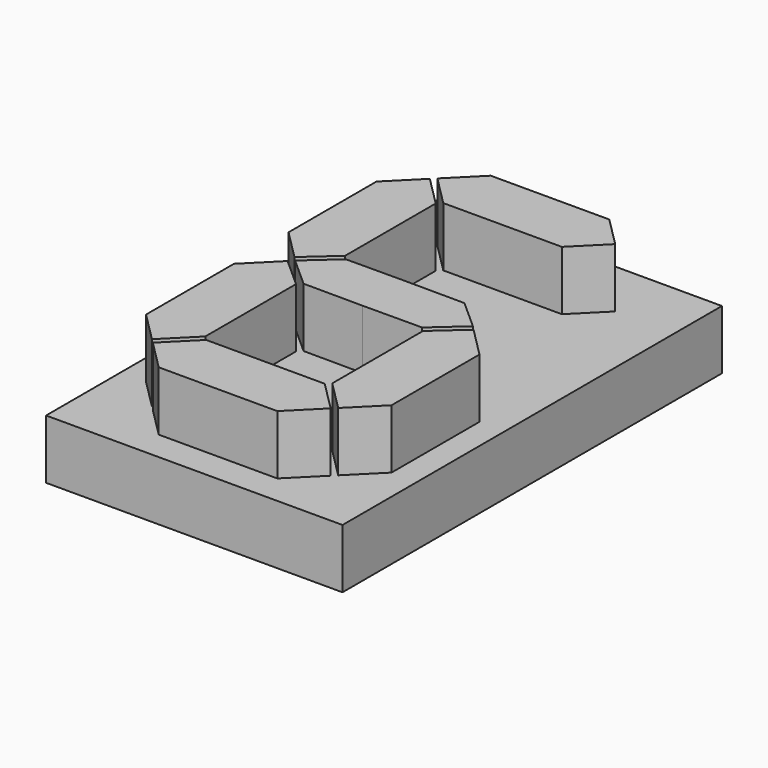
from build123d import *

# Parameters (mm, degrees)
F0_W     = 10
F0_H     = 16
F1_DEPTH = 2
F3_DEPTH = 2


# Not quite as in the source:
# - ends of sketch curves that miss each other by under 0.0002 mm in the source are joined
# - a feature names something its author has since deleted; it is built from what else it names


with BuildPart() as f1:
    # F0 (on Top) → F1 (new body)
    with BuildSketch(Plane.XY):
        Rectangle(F0_W, F0_H)
    extrude(amount=F1_DEPTH)

    # F2 (on face) → F3 (join)
    with BuildSketch(Plane.XY.offset(2)):
        Polygon((0, 7), (-2, 7), (-3, 6), (-2, 5), (0, 5), (2, 5), (3, 6), (2, 7), align=None)
        Polygon((-2.1414213562, 4.8585786438), (-3.1414213562, 5.8585786438), (-4.1414213562, 4.8585786438), (-4.1414213562, 1.1507223826), (-3.1374518146, 0.1453992321), (-2.1414213562, 1.0335195075), align=None)
        Polygon((2, 0.891659756), (2.00782e-05, 0.9006214721), (-2, 0.891659756), (-3, 0), (-2, -0.891659756), (-2.00782e-05, -0.9006214721), (2, -0.891659756), (3, 0), align=None)
        Polygon((3.1374518146, -0.1453992321), (2.1414213562, -1.0335195075), (2.1414213562, -4.8585786438), (3.1414213562, -5.8585786438), (4.1414213562, -4.8585786438), (4.1414213562, -1.1507223826), align=None)
        Polygon((0, -5), (-2, -5), (-3, -6), (-2, -7), (0, -7), (2, -7), (3, -6), (2, -5), align=None)
        Polygon((-4.1414213562, -4.8585786438), (-3.1414213562, -5.8585786438), (-2.1414213562, -4.8585786438), (-2.1414213562, -1.0335195075), (-3.1374518146, -0.1453992321), (-4.1414213562, -1.1507223826), align=None)
    extrude(amount=F3_DEPTH)


solid = f1.part
